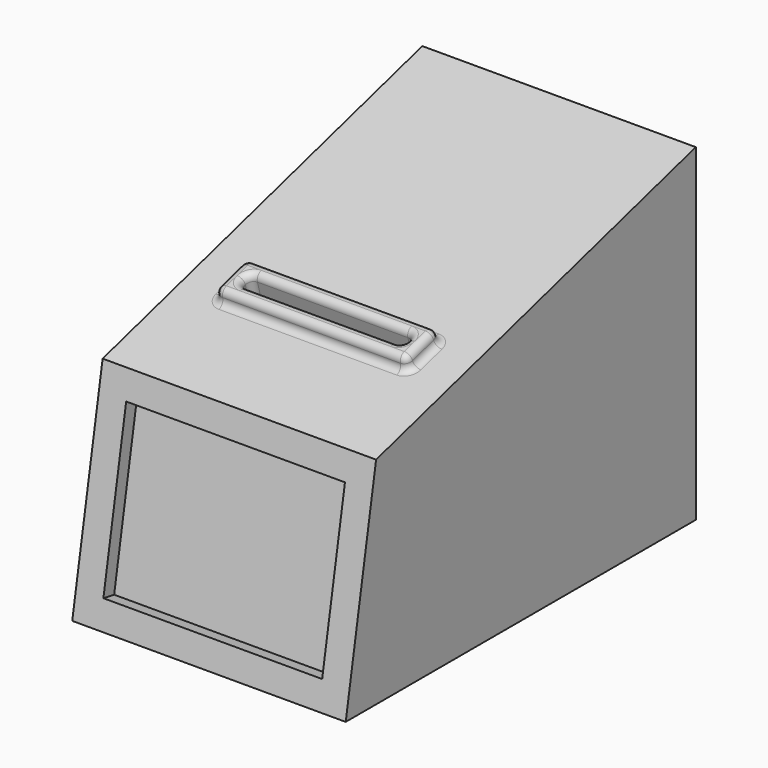
from build123d import *

# Parameters (mm, degrees)
F1_DEPTH = 127
F2_W     = 101.6
F2_H     = 76.2
F3_DEPTH = 6.35
F4_W     = 76.2
F4_H     = 6.35
F5_DEPTH = 25.4
F7_DEPTH = 6.35
F8_R     = 3.17499
F9_R     = 3.17499


# Not quite as in the source:
# - a fillet or chamfer is up to 0.001 mm smaller than in the source, because OpenCascade refuses the exact size


with BuildPart() as f1:
    # F0 (on Right) → F1 (new body)
    with BuildSketch(Plane.YZ):
        Polygon((-65.1389909149, 110.2977480159), (-82.7816457659, 10.2412803099), (120.4183542341, 10.2412803099), (120.4183542341, 162.6412803099), align=None)
    extrude(amount=F1_DEPTH)

    # F2 (on face) → F3 (cut)
    with BuildSketch(Plane(origin=(0, -82.036835794, 14.4653075624), x_dir=(1, 0, 0), z_dir=(0, -0.984807753, 0.1736481777))):
        with Locations((63.5, 46.5108103184)):
            Rectangle(F2_W, F2_H)
    extrude(amount=-F3_DEPTH, mode=Mode.SUBTRACT)

    # F4 (on face) → F5 (cut)
    with BuildSketch(Plane(origin=(0, -33.6216432412, 119.1884190074), x_dir=(1, 0, 0), z_dir=(0, -0.2714930529, 0.9624403993))):
        with Locations((63.5, 21.2276759098)):
            Rectangle(F4_W, F4_H)
    extrude(amount=-F5_DEPTH, mode=Mode.SUBTRACT)

    # F6 (on face) → F7 (join)
    with BuildSketch(Plane(origin=(0, -33.6216432412, 119.1884190074), x_dir=(1, 0, 0), z_dir=(0, -0.2714930529, 0.9624403993))):
        Polygon((25.4, 30.7526759098), (25.4, 24.4026759098), (101.6, 24.4026759098), (101.6, 18.0526759098), (101.6, 11.7026759098), (107.95, 11.7026759098), (107.95, 30.7526759098), align=None)
        Polygon((25.4, 18.0526759098), (25.4, 24.4026759098), (25.4, 30.7526759098), (19.05, 30.7526759098), (19.05, 11.7026759098), (101.6, 11.7026759098), (101.6, 18.0526759098), align=None)
    extrude(amount=F7_DEPTH)

    # F8 (radius 3.175 in the source; OpenCascade refuses exactly that, so slightly less here)
    f8_edges = [f1.edges().sort_by_distance(p)[0] for p in [
        (63.5, -22.358515, 122.365614),
        (107.95, -13.19127, 124.951586),
        (63.5, -4.024026, 127.537557),
        (19.05, -13.19127, 124.951586),
        (63.5, -24.082496, 128.477111),
        (107.95, -14.915251, 131.063082),
        (63.5, -5.748006, 133.649053),
        (19.05, -14.915251, 131.063082),
        (19.05, -23.220506, 125.421362),
        (19.05, -4.886016, 130.593305),
        (107.95, -23.220506, 125.421362),
        (107.95, -4.886016, 130.593305),
        (63.5, -11.859503, 131.925073),
        (101.6, -14.915251, 131.063082),
        (63.5, -17.971, 130.201092),
        (25.4, -14.915251, 131.063082),
        (25.4, -13.661047, 114.92235),
        (25.4, -7.549551, 116.646331),
        (101.6, -7.549551, 116.646331),
        (101.6, -13.661047, 114.92235),
    ]]
    fillet(f8_edges, radius=F8_R)

    # F9 (radius 3.175 in the source; OpenCascade refuses exactly that, so slightly less here)
    f9_edges = [f1.edges().sort_by_distance(p)[0] for p in [
        (63.5, -3.239599, 101.36759),
    ]]
    fillet(f9_edges, radius=F9_R)


solid = f1.part
